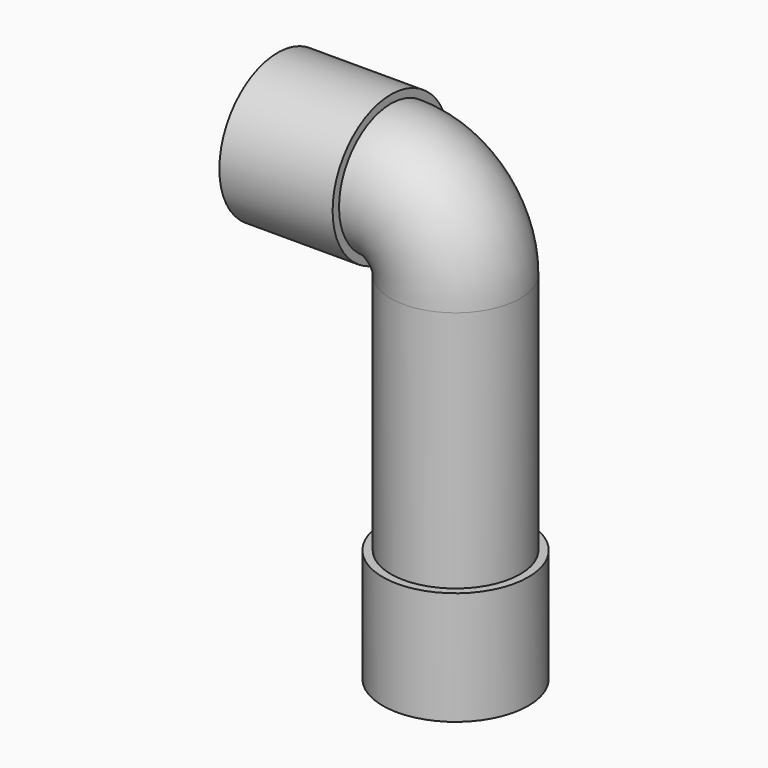
from build123d import *

# Parameters (mm, degrees)
F1_R     = 20
F3_R     = 22.5
F4_DEPTH = 35
F5_R     = 22.5
F5_R_2   = 20
F6_DEPTH = 35
F7_DEPTH = 30


with BuildPart() as f2:
    # F2: sweep along a path in F0
    with BuildLine(Plane.XZ) as f2_path:
        ThreePointArc((-20, 130), (-5.8578643763, 124.1421356237), (0, 110))
        Line((0, 110), (0, 0))
    # F1 (on Top) → F2 (sweep)
    with BuildSketch(Plane.XY):
        Circle(F1_R)
    sweep(path=f2_path.line)

    # F3 (on Top) → F4 (join)
    with BuildSketch(Plane.XY):
        Circle(F3_R)
    extrude(amount=F4_DEPTH)


with BuildPart() as f6:
    # F5 (on face) → F6 (new body)
    with BuildSketch(Plane(origin=(-20, 0, 0), x_dir=(0, -1, 0), z_dir=(-1, 0, 0))):
        with Locations((0, 130)):
            Circle(F5_R)
        with Locations((0, 130)):
            Circle(F5_R_2, mode=Mode.SUBTRACT)
    extrude(amount=F6_DEPTH)


with BuildPart() as f7:
    # F7 (new): a face of the model
    f7_faces = [f2.part.faces().sort_by_distance(p)[0] for p in [
        (-20, 0, 130),
    ]]
    extrude(f7_faces, amount=F7_DEPTH)


solid = Compound([f2.part, f6.part, f7.part])
